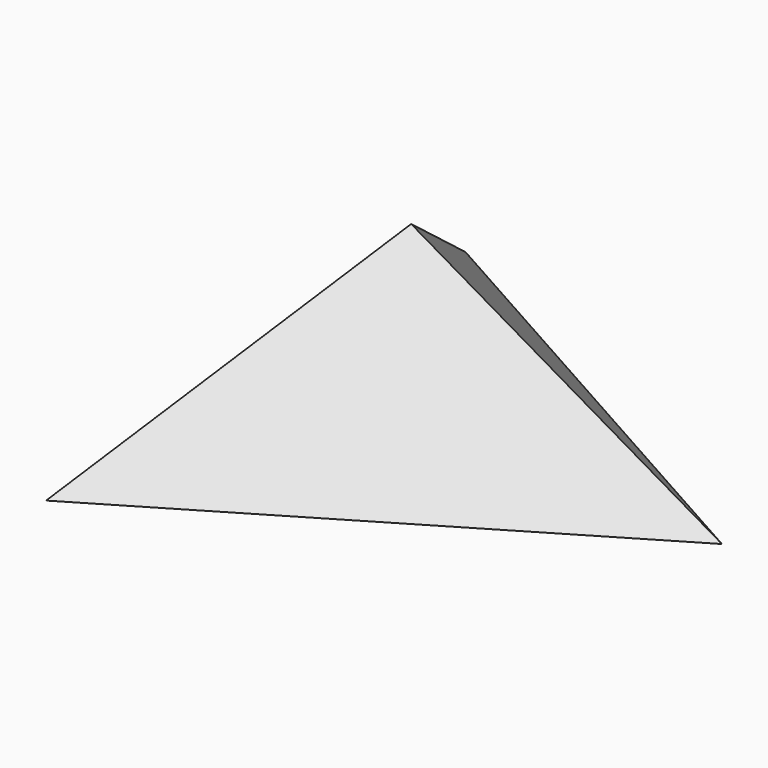
from build123d import *

# Parameters (mm, degrees)
F1_DEPTH     = 30
F1_TAPER     = 40
F3_R         = 10
F4_DEPTH     = 5
F2_TEXT_SIZE = 5.1208040936
F5_DEPTH     = 2


# Not quite as in the source:
# - Text() gives the source's letters only with a copy of the font that has no kerning and outlines rounded to 1/6400 em; it was checked with that copy


with BuildPart() as f1:
    # F0 (on Top) → F1 (new body)
    with BuildSketch(Plane.XY):
        Polygon((28.8651575945, 0.3687958453), (-14.7519653681, 24.8135618385), (-14.1131922264, -25.1823576838), align=None)
    extrude(amount=F1_DEPTH, taper=F1_TAPER)

    # F3 (on face) → F4 (cut)
    with BuildSketch(Plane(origin=(0, 0, 0), x_dir=(1, 0, 0), z_dir=(0, 0, -1))):
        Circle(F3_R)
    extrude(amount=-F4_DEPTH, mode=Mode.SUBTRACT)

    # F2 (on face) → F5 (cut)
    with BuildSketch(Plane(origin=(-8.4693849022, -0.1082091429, 7.1072377663), x_dir=(0.0074966965, -0.9999521104, -0.0062909887), z_dir=(-0.7659819266, -0.0097865723, 0.6427876097))):
        with Locations((-13.3877554908, -6.3179745339)):
            Text('OsirisZero', F2_TEXT_SIZE, font='Open Sans', text_align=(TextAlign.LEFT, TextAlign.BOTTOM))
    extrude(amount=-F5_DEPTH, mode=Mode.SUBTRACT)


solid = f1.part
